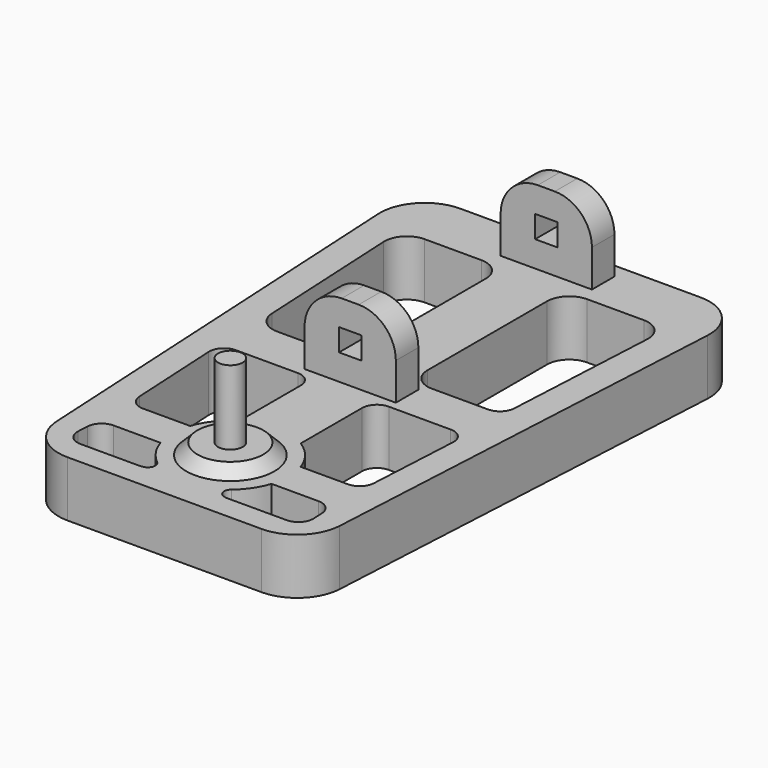
from build123d import *

# Parameters (mm, degrees)
F1_DEPTH     = 19.05
F2_R         = 15.059033574
F3_DEPTH     = 3.81
F6_DEPTH     = 25.4
F8_DEPTH     = 98.4172728563
F4_R         = 4.2206847971
F9_DEPTH     = 25.4
F10_SIZE     = 3.80999
F11_R        = 12.7
F12_R        = 12.7
F13_R        = 7.62
F14_R        = 5.08
F15_R        = 7.62
F16_R        = 7.62
F17_R        = 5.08
F18_R        = 7.62
F19_R        = 5.08
F20_T1_DEPTH = 19.05
F21_R        = 2.54
F22_R        = 15.24


# Not quite as in the source:
# - a fillet or chamfer that OpenCascade refuses, or shapes differently, is made with other operations: its cross-section is extruded or revolved along the edge and cut away or added
# - a fillet or chamfer is up to 0.001 mm smaller than in the source, because OpenCascade refuses the exact size


with BuildPart() as f1:
    # F0 (on Top) → F1 (new body)
    with BuildSketch(Plane.XY):
        Polygon((57.15, 90.8419879414), (0, 90.8419879414), (-57.15, 90.8419879414), (-47.625, -86.9580120586), (0, -86.9580120586), (47.625, -86.9580120586), align=None)
        with BuildLine():
            Line((-39.8510134111, -64.9218410254), (-19.0060128585, -64.9218410254))
            ThreePointArc((-19.0060128585, -64.9218410254), (-15.7100075961, -71.1253052436), (-10.4695623741, -75.8033767343))
            Line((-10.4695623741, -75.8033767343), (-10.4695623741, -78.8165818754))
            Line((-10.4695623741, -78.8165818754), (-40.5953745281, -78.8165818754))
            Line((-40.5953745281, -78.8165818754), (-39.8510134111, -64.9218410254))
        make_face(mode=Mode.SUBTRACT)
        with BuildLine():
            Line((-42.0940332115, -10.5141438544), (-10.4695623741, -10.5141438544))
            Line((-10.4695623741, -10.5141438544), (-10.4695623741, -41.7985618114))
            ThreePointArc((-10.4695623741, -41.7985618114), (-15.6132317705, -46.3542592872), (-18.9080441845, -52.3838467943))
            Line((-18.9080441845, -52.3838467943), (-39.8510134111, -52.3838467943))
            Line((-39.8510134111, -52.3838467943), (-42.0940332115, -10.5141438544))
        make_face(mode=Mode.SUBTRACT)
        with BuildLine():
            Line((19.0060128585, -64.9218410254), (39.8510134111, -64.9218410254))
            Line((39.8510134111, -64.9218410254), (40.5953745281, -78.8165818754))
            Line((40.5953745281, -78.8165818754), (10.4695623741, -78.8165818754))
            Line((10.4695623741, -78.8165818754), (10.4695623741, -75.8033767343))
            ThreePointArc((10.4695623741, -75.8033767343), (15.7100075961, -71.1253052436), (19.0060128585, -64.9218410254))
        make_face(mode=Mode.SUBTRACT)
        with BuildLine():
            Line((10.4695623741, -10.5141438544), (42.0940332115, -10.5141438544))
            Line((42.0940332115, -10.5141438544), (39.8510134111, -52.3838467943))
            Line((39.8510134111, -52.3838467943), (18.9080441845, -52.3838467943))
            ThreePointArc((18.9080441845, -52.3838467943), (15.6132317705, -46.3542592872), (10.4695623741, -41.7985618114))
            Line((10.4695623741, -41.7985618114), (10.4695623741, -10.5141438544))
        make_face(mode=Mode.SUBTRACT)
        Polygon((-10.4695623741, 71.0973963141), (-10.4695623741, 4.7880196944), (-42.0940332115, 4.7880196944), (-45.4945191741, 71.0973963141), align=None, mode=Mode.SUBTRACT)
        Polygon((10.4695623741, 4.7880196944), (10.4695623741, 71.0973963141), (45.4945191741, 71.0973963141), (42.0940332115, 4.7880196944), align=None, mode=Mode.SUBTRACT)
    extrude(amount=F1_DEPTH)

    # F2 (on face) → F3 (join)
    with BuildSketch(Plane.XY.offset(19.05)):
        with Locations((0, -58.8009692729)):
            Circle(F2_R)
    extrude(amount=F3_DEPTH)

    # F5 (on face) → F6 (join)
    with BuildSketch(Plane.XY.offset(19.05)):
        Polygon((15.6109640375, 85.8776420355), (0, 85.8776420355), (-15.6109640375, 85.8776420355), (-15.6109640375, 76.2544423342), (0, 76.2544423342), (15.6109640375, 76.2544423342), align=None)
        Polygon((-15.6109640375, -7.5742849149), (0, -7.5742849149), (15.6109640375, -7.5742849149), (15.6109640375, 2.0489108283), (0, 2.0489108283), (-15.6109640375, 2.0489108283), align=None)
    extrude(amount=F6_DEPTH)

    # F7 (on face) → F8 (cut, through all)
    with BuildSketch(Plane.XZ.offset(7.5742849149)):
        Polygon((3.81, 35.5143319389), (0, 35.5143319389), (-3.81, 35.5143319389), (-3.81, 27.8943319389), (0, 27.8943319389), (3.81, 27.8943319389), align=None)
    extrude(amount=-F8_DEPTH, mode=Mode.SUBTRACT)

    # F4 (on face) → F9 (join)
    with BuildSketch(Plane.XY.offset(22.86)):
        with Locations((0, -58.8009692729)):
            Circle(F4_R)
    extrude(amount=F9_DEPTH)

    # F10 (size 3.81 in the source; OpenCascade refuses exactly that, so slightly less here)
    f10_edges = [f1.edges().sort_by_distance(p)[0] for p in [
        (-15.059034, -58.800969, 22.86),
    ]]
    chamfer(f10_edges, length=F10_SIZE)

    # F11
    f11_edges = [f1.edges().sort_by_distance(p)[0] for p in [
        (15.610964, -2.762687, 44.45),
        (-15.610964, -2.762687, 44.45),
    ]]
    fillet(f11_edges, radius=F11_R)

    # F12
    f12_edges = [f1.edges().sort_by_distance(p)[0] for p in [
        (15.610964, 81.066042, 44.45),
        (-15.610964, 81.066042, 44.45),
    ]]
    fillet(f12_edges, radius=F12_R)

    # F13
    f13_edges = [f1.edges().sort_by_distance(p)[0] for p in [
        (-45.494519, 71.097396, 9.525),
    ]]
    fillet(f13_edges, radius=F13_R)

    # F14
    f14_edges = [f1.edges().sort_by_distance(p)[0] for p in [
        (-42.094033, -10.514144, 9.525),
    ]]
    fillet(f14_edges, radius=F14_R)

    # F15
    f15_edges = [f1.edges().sort_by_distance(p)[0] for p in [
        (-10.469562, 71.097396, 9.525),
        (45.494519, 71.097396, 9.525),
    ]]
    fillet(f15_edges, radius=F15_R)

    # F16
    f16_edges = [f1.edges().sort_by_distance(p)[0] for p in [
        (-42.094033, 4.78802, 9.525),
        (10.469562, 4.78802, 9.525),
    ]]
    fillet(f16_edges, radius=F16_R)

    # F17
    f17_edges = [f1.edges().sort_by_distance(p)[0] for p in [
        (-10.469562, 4.78802, 9.525),
        (42.094033, 4.78802, 9.525),
    ]]
    fillet(f17_edges, radius=F17_R)

    # F18
    f18_edges = [f1.edges().sort_by_distance(p)[0] for p in [
        (10.469562, 71.097396, 9.525),
    ]]
    fillet(f18_edges, radius=F18_R)

    # F19
    f19_edges = [f1.edges().sort_by_distance(p)[0] for p in [
        (-10.469562, -10.514144, 9.525),
        (42.094033, -10.514144, 9.525),
        (10.469562, -10.514144, 9.525),
        (-39.851013, -52.383847, 9.525),
        (39.851013, -52.383847, 9.525),
    ]]
    fillet(f19_edges, radius=F19_R)

    # F20: fillet of radius 5.08 on 6 edges, made by hand

    # F20_s2 → F20_t1 (join)
    with BuildSketch(Plane.XY):
        with BuildLine():
            ThreePointArc((40.3086734646, -73.4648286909), (38.9228773885, -77.2312845683), (35.2359473527, -78.8165818754))
            Line((35.2359473527, -78.8165818754), (40.5953745281, -78.8165818754))
            Line((40.5953745281, -78.8165818754), (40.3086734646, -73.4648286909))
        make_face()
        with BuildLine():
            ThreePointArc((-15.1101182687, -78.8165818754), (-12.3436148694, -77.9971990774), (-10.4695623741, -75.8033767343))
            Line((-10.4695623741, -75.8033767343), (-10.4695623741, -78.8165818754))
            Line((-10.4695623741, -78.8165818754), (-15.1101182687, -78.8165818754))
        make_face()
        with BuildLine():
            ThreePointArc((-40.3086734646, -73.4648286909), (-38.9228773885, -77.2312845683), (-35.2359473527, -78.8165818754))
            Line((-35.2359473527, -78.8165818754), (-40.5953745281, -78.8165818754))
            Line((-40.5953745281, -78.8165818754), (-40.3086734646, -73.4648286909))
        make_face()
        with BuildLine():
            ThreePointArc((10.4695623741, -75.8033767343), (12.3436148694, -77.9971990774), (15.1101182687, -78.8165818754))
            Line((15.1101182687, -78.8165818754), (10.4695623741, -78.8165818754))
            Line((10.4695623741, -78.8165818754), (10.4695623741, -75.8033767343))
        make_face()
        with BuildLine():
            ThreePointArc((35.03587195, -64.9218410254), (38.5305746428, -66.3149109896), (40.1085980619, -69.7300878408))
            Line((40.1085980619, -69.7300878408), (39.8510134111, -64.9218410254))
            Line((39.8510134111, -64.9218410254), (35.03587195, -64.9218410254))
        make_face()
        with BuildLine():
            ThreePointArc((-35.03587195, -64.9218410254), (-38.5305746428, -66.3149109896), (-40.1085980619, -69.7300878408))
            Line((-40.1085980619, -69.7300878408), (-39.8510134111, -64.9218410254))
            Line((-39.8510134111, -64.9218410254), (-35.03587195, -64.9218410254))
        make_face()
    extrude(amount=F20_T1_DEPTH)

    # F21
    f21_edges = [f1.edges().sort_by_distance(p)[0] for p in [
        (10.469562, -75.803377, 9.525),
        (-10.469562, -75.803377, 9.525),
    ]]
    fillet(f21_edges, radius=F21_R)

    # F22
    f22_edges = [f1.edges().sort_by_distance(p)[0] for p in [
        (-47.625, -86.958012, 9.525),
        (-57.15, 90.841988, 9.525),
        (57.15, 90.841988, 9.525),
        (47.625, -86.958012, 9.525),
    ]]
    fillet(f22_edges, radius=F22_R)


solid = f1.part
